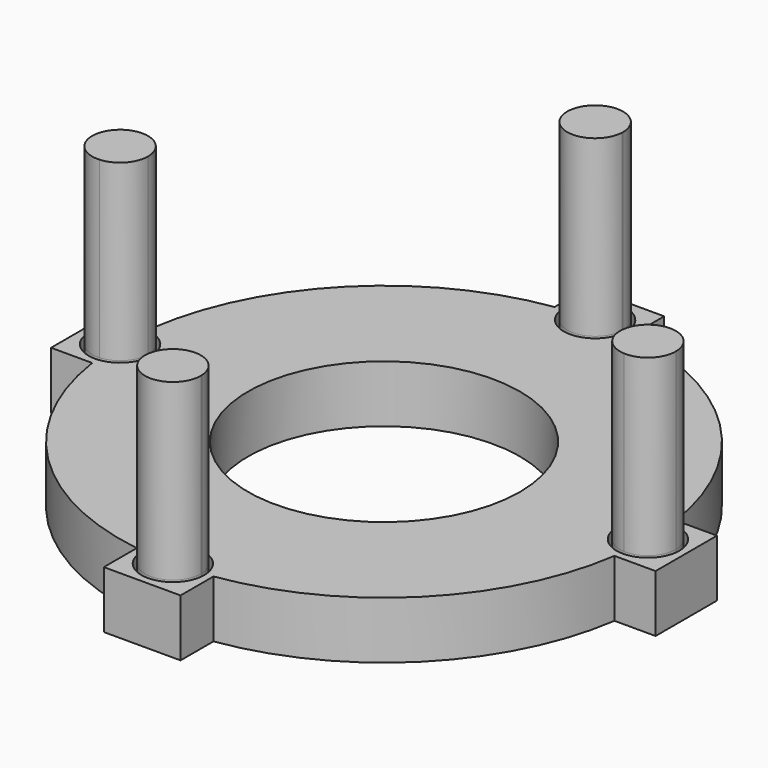
from build123d import *

# Parameters (mm, degrees)
F0_R     = 20
F0_R_2   = 19.5
F1_DEPTH = 8.2
F3_DEPTH = 25


# Not quite as in the source:
# - the program builds the solid bodies; features that only make, move or delete a surface that nothing else refers to are left out


with BuildPart() as f1:
    # F0 (on Top) → F1 (new body)
    with BuildSketch(Plane.XY):
        with BuildLine():
            ThreePointArc((37.5774613555, -4.492039968), (33.345, 0), (37.5774613555, 4.492039968))
            ThreePointArc((37.5774613555, 4.492039968), (37.5137215364, 4.9964709038), (37.4432106663, 5.5))
            Line((37.4432106663, 5.5), (32.345, 5.5))
            Line((32.345, 5.5), (32.345, -5.5))
            Line((32.345, -5.5), (37.4432106663, -5.5))
            ThreePointArc((37.4432106663, -5.5), (37.5137215364, -4.9964709038), (37.5774613555, -4.492039968))
        make_face()
        with BuildLine():
            ThreePointArc((37.4432106663, 5.5), (37.5137215364, 4.9964709038), (37.5774613555, 4.492039968))
            ThreePointArc((37.5774613555, 4.492039968), (40.9309420037, 3.2752041082), (42.345, 0))
            ThreePointArc((42.345, 0), (40.9309420037, -3.2752041082), (37.5774613555, -4.492039968))
            ThreePointArc((37.5774613555, -4.492039968), (37.5137215364, -4.9964709038), (37.4432106663, -5.5))
            Line((37.4432106663, -5.5), (43.345, -5.5))
            Line((43.345, -5.5), (43.345, 5.5))
            Line((43.345, 5.5), (37.4432106663, 5.5))
        make_face()
        with BuildLine():
            Line((32.345, 5.5), (37.4432106663, 5.5))
            ThreePointArc((37.4432106663, 5.5), (26.760456134, 26.760456134), (5.5, 37.4432106663))
            Line((5.5, 37.4432106663), (5.5, 32.345))
            Line((5.5, 32.345), (-5.5, 32.345))
            Line((-5.5, 32.345), (-5.5, 37.4432106663))
            ThreePointArc((-5.5, 37.4432106663), (-26.760456134, 26.760456134), (-37.4432106663, 5.5))
            Line((-37.4432106663, 5.5), (-32.345, 5.5))
            Line((-32.345, 5.5), (-32.345, -5.5))
            Line((-32.345, -5.5), (-37.4432106663, -5.5))
            ThreePointArc((-37.4432106663, -5.5), (-26.760456134, -26.760456134), (-5.5, -37.4432106663))
            Line((-5.5, -37.4432106663), (-5.5, -32.345))
            Line((-5.5, -32.345), (5.5, -32.345))
            Line((5.5, -32.345), (5.5, -37.4432106663))
            ThreePointArc((5.5, -37.4432106663), (26.760456134, -26.760456134), (37.4432106663, -5.5))
            Line((37.4432106663, -5.5), (32.345, -5.5))
            Line((32.345, -5.5), (32.345, 5.5))
        make_face()
        with BuildLine():
            ThreePointArc((23.3205760812, 16.9760053087), (27.4291454667, 8.9261416059), (28.845, 0))
            ThreePointArc((28.845, 0), (27.4291454667, -8.9261416059), (23.3205760812, -16.9760053087))
            ThreePointArc((23.3205760812, -16.9760053087), (24.483570121, -18.5134609029), (24.8964951033, -20.3964951033))
            ThreePointArc((24.8964951033, -20.3964951033), (21.9549873112, -24.6179998158), (16.9760053087, -23.3205760812))
            ThreePointArc((16.9760053087, -23.3205760812), (0, -28.845), (-16.9760053087, -23.3205760812))
            ThreePointArc((-16.9760053087, -23.3205760812), (-23.5784756187, -23.5784756187), (-23.3205760812, -16.9760053087))
            ThreePointArc((-23.3205760812, -16.9760053087), (-28.845, 0), (-23.3205760812, 16.9760053087))
            ThreePointArc((-23.3205760812, 16.9760053087), (-23.5784756187, 23.5784756187), (-16.9760053087, 23.3205760812))
            ThreePointArc((-16.9760053087, 23.3205760812), (0, 28.845), (16.9760053087, 23.3205760812))
            ThreePointArc((16.9760053087, 23.3205760812), (21.9549873112, 24.6179998158), (24.8964951033, 20.3964951033))
            ThreePointArc((24.8964951033, 20.3964951033), (24.483570121, 18.5134609029), (23.3205760812, 16.9760053087))
        make_face(mode=Mode.SUBTRACT)
        with BuildLine():
            Line((5.5, 32.345), (5.5, 37.4432106663))
            ThreePointArc((5.5, 37.4432106663), (4.9964709038, 37.5137215364), (4.492039968, 37.5774613555))
            ThreePointArc((4.492039968, 37.5774613555), (0, 33.345), (-4.492039968, 37.5774613555))
            ThreePointArc((-4.492039968, 37.5774613555), (-4.9964709038, 37.5137215364), (-5.5, 37.4432106663))
            Line((-5.5, 37.4432106663), (-5.5, 32.345))
            Line((-5.5, 32.345), (5.5, 32.345))
        make_face()
        with BuildLine():
            ThreePointArc((4.492039968, 37.5774613555), (4.9964709038, 37.5137215364), (5.5, 37.4432106663))
            Line((5.5, 37.4432106663), (5.5, 43.345))
            Line((5.5, 43.345), (-5.5, 43.345))
            Line((-5.5, 43.345), (-5.5, 37.4432106663))
            ThreePointArc((-5.5, 37.4432106663), (-4.9964709038, 37.5137215364), (-4.492039968, 37.5774613555))
            ThreePointArc((-4.492039968, 37.5774613555), (-0.1338285175, 42.3430095518), (4.5, 37.845))
            ThreePointArc((4.5, 37.845), (4.4980095518, 37.7111714825), (4.492039968, 37.5774613555))
        make_face()
        with BuildLine():
            Line((5.5, -43.345), (5.5, -37.4432106663))
            ThreePointArc((5.5, -37.4432106663), (4.9964709038, -37.5137215364), (4.492039968, -37.5774613555))
            ThreePointArc((4.492039968, -37.5774613555), (4.4980095518, -37.7111714825), (4.5, -37.845))
            ThreePointArc((4.5, -37.845), (-0.1338285175, -42.3430095518), (-4.492039968, -37.5774613555))
            ThreePointArc((-4.492039968, -37.5774613555), (-4.9964709038, -37.5137215364), (-5.5, -37.4432106663))
            Line((-5.5, -37.4432106663), (-5.5, -43.345))
            Line((-5.5, -43.345), (5.5, -43.345))
        make_face()
        with BuildLine():
            ThreePointArc((4.492039968, -37.5774613555), (4.9964709038, -37.5137215364), (5.5, -37.4432106663))
            Line((5.5, -37.4432106663), (5.5, -32.345))
            Line((5.5, -32.345), (-5.5, -32.345))
            Line((-5.5, -32.345), (-5.5, -37.4432106663))
            ThreePointArc((-5.5, -37.4432106663), (-4.9964709038, -37.5137215364), (-4.492039968, -37.5774613555))
            ThreePointArc((-4.492039968, -37.5774613555), (0, -33.345), (4.492039968, -37.5774613555))
        make_face()
        with BuildLine():
            Line((-32.345, 5.5), (-37.4432106663, 5.5))
            ThreePointArc((-37.4432106663, 5.5), (-37.5137215364, 4.9964709038), (-37.5774613555, 4.492039968))
            ThreePointArc((-37.5774613555, 4.492039968), (-34.5697958918, 3.0859420037), (-33.345, 0))
            ThreePointArc((-33.345, 0), (-34.5697958918, -3.0859420037), (-37.5774613555, -4.492039968))
            ThreePointArc((-37.5774613555, -4.492039968), (-37.5137215364, -4.9964709038), (-37.4432106663, -5.5))
            Line((-37.4432106663, -5.5), (-32.345, -5.5))
            Line((-32.345, -5.5), (-32.345, 5.5))
        make_face()
        with BuildLine():
            ThreePointArc((-37.5774613555, 4.492039968), (-37.5137215364, 4.9964709038), (-37.4432106663, 5.5))
            Line((-37.4432106663, 5.5), (-43.345, 5.5))
            Line((-43.345, 5.5), (-43.345, -5.5))
            Line((-43.345, -5.5), (-37.4432106663, -5.5))
            ThreePointArc((-37.4432106663, -5.5), (-37.5137215364, -4.9964709038), (-37.5774613555, -4.492039968))
            ThreePointArc((-37.5774613555, -4.492039968), (-42.345, 0), (-37.5774613555, 4.492039968))
        make_face()
        with BuildLine():
            ThreePointArc((-23.3205760812, 16.9760053087), (-20.3964951033, 20.3964951033), (-16.9760053087, 23.3205760812))
            ThreePointArc((-16.9760053087, 23.3205760812), (-23.5784756187, 23.5784756187), (-23.3205760812, 16.9760053087))
        make_face()
        with BuildLine():
            ThreePointArc((16.9760053087, 23.3205760812), (20.3964951033, 20.3964951033), (23.3205760812, 16.9760053087))
            ThreePointArc((23.3205760812, 16.9760053087), (24.483570121, 18.5134609029), (24.8964951033, 20.3964951033))
            ThreePointArc((24.8964951033, 20.3964951033), (21.9549873112, 24.6179998158), (16.9760053087, 23.3205760812))
        make_face()
        with BuildLine():
            ThreePointArc((24.8964951033, -20.3964951033), (24.483570121, -18.5134609029), (23.3205760812, -16.9760053087))
            ThreePointArc((23.3205760812, -16.9760053087), (20.3964951033, -20.3964951033), (16.9760053087, -23.3205760812))
            ThreePointArc((16.9760053087, -23.3205760812), (21.9549873112, -24.6179998158), (24.8964951033, -20.3964951033))
        make_face()
        with BuildLine():
            ThreePointArc((-23.3205760812, -16.9760053087), (-23.5784756187, -23.5784756187), (-16.9760053087, -23.3205760812))
            ThreePointArc((-16.9760053087, -23.3205760812), (-20.3964951033, -20.3964951033), (-23.3205760812, -16.9760053087))
        make_face()
        with BuildLine():
            ThreePointArc((23.3205760812, -16.9760053087), (27.4291454667, -8.9261416059), (28.845, 0))
            ThreePointArc((28.845, 0), (27.4291454667, 8.9261416059), (23.3205760812, 16.9760053087))
            ThreePointArc((23.3205760812, 16.9760053087), (17.214514588, 17.214514588), (16.9760053087, 23.3205760812))
            ThreePointArc((16.9760053087, 23.3205760812), (0, 28.845), (-16.9760053087, 23.3205760812))
            ThreePointArc((-16.9760053087, 23.3205760812), (-16.1749903908, 21.9549873112), (-15.8964951033, 20.3964951033))
            ThreePointArc((-15.8964951033, 20.3964951033), (-18.5134609029, 16.3094200856), (-23.3205760812, 16.9760053087))
            ThreePointArc((-23.3205760812, 16.9760053087), (-28.845, 0), (-23.3205760812, -16.9760053087))
            ThreePointArc((-23.3205760812, -16.9760053087), (-18.5134609029, -16.3094200856), (-15.8964951033, -20.3964951033))
            ThreePointArc((-15.8964951033, -20.3964951033), (-16.1749903908, -21.9549873112), (-16.9760053087, -23.3205760812))
            ThreePointArc((-16.9760053087, -23.3205760812), (0, -28.845), (16.9760053087, -23.3205760812))
            ThreePointArc((16.9760053087, -23.3205760812), (17.214514588, -17.214514588), (23.3205760812, -16.9760053087))
        make_face()
        Circle(F0_R, mode=Mode.SUBTRACT)
        with BuildLine():
            ThreePointArc((16.9760053087, -23.3205760812), (20.3964951033, -20.3964951033), (23.3205760812, -16.9760053087))
            ThreePointArc((23.3205760812, -16.9760053087), (17.214514588, -17.214514588), (16.9760053087, -23.3205760812))
        make_face()
        with BuildLine():
            ThreePointArc((16.9760053087, 23.3205760812), (17.214514588, 17.214514588), (23.3205760812, 16.9760053087))
            ThreePointArc((23.3205760812, 16.9760053087), (20.3964951033, 20.3964951033), (16.9760053087, 23.3205760812))
        make_face()
        with BuildLine():
            ThreePointArc((-15.8964951033, 20.3964951033), (-16.1749903908, 21.9549873112), (-16.9760053087, 23.3205760812))
            ThreePointArc((-16.9760053087, 23.3205760812), (-20.3964951033, 20.3964951033), (-23.3205760812, 16.9760053087))
            ThreePointArc((-23.3205760812, 16.9760053087), (-18.5134609029, 16.3094200856), (-15.8964951033, 20.3964951033))
        make_face()
        with BuildLine():
            ThreePointArc((-23.3205760812, -16.9760053087), (-20.3964951033, -20.3964951033), (-16.9760053087, -23.3205760812))
            ThreePointArc((-16.9760053087, -23.3205760812), (-16.1749903908, -21.9549873112), (-15.8964951033, -20.3964951033))
            ThreePointArc((-15.8964951033, -20.3964951033), (-18.5134609029, -16.3094200856), (-23.3205760812, -16.9760053087))
        make_face()
        Circle(F0_R)
        Circle(F0_R_2, mode=Mode.SUBTRACT)
    extrude(amount=F1_DEPTH)


with BuildPart() as f1b:
    # F0 (on Top) → F1, piece 2 (new body)
    with BuildSketch(Plane.XY):
        with BuildLine():
            ThreePointArc((-37.6336114414, -3.9944104543), (-37.845, 0), (-37.6336114414, 3.9944104543))
            ThreePointArc((-37.6336114414, 3.9944104543), (-41.845, 0), (-37.6336114414, -3.9944104543))
        make_face()
        with BuildLine():
            ThreePointArc((-33.845, 0), (-34.9427978848, 2.7526755862), (-37.6336114414, 3.9944104543))
            ThreePointArc((-37.6336114414, 3.9944104543), (-37.845, 0), (-37.6336114414, -3.9944104543))
            ThreePointArc((-37.6336114414, -3.9944104543), (-34.9427978848, -2.7526755862), (-33.845, 0))
        make_face()
    extrude(amount=F1_DEPTH)


with BuildPart() as f1c:
    # F0 (on Top) → F1, piece 3 (new body)
    with BuildSketch(Plane.XY):
        with BuildLine():
            ThreePointArc((-3.9944104543, 37.6336114414), (0, 37.845), (3.9944104543, 37.6336114414))
            ThreePointArc((3.9944104543, 37.6336114414), (3.9986023694, 37.7392687774), (4, 37.845))
            ThreePointArc((4, 37.845), (-0.1057312226, 41.8436023694), (-3.9944104543, 37.6336114414))
        make_face()
        with BuildLine():
            ThreePointArc((-3.9944104543, 37.6336114414), (0, 33.845), (3.9944104543, 37.6336114414))
            ThreePointArc((3.9944104543, 37.6336114414), (0, 37.845), (-3.9944104543, 37.6336114414))
        make_face()
    extrude(amount=F1_DEPTH)


with BuildPart() as f1d:
    # F0 (on Top) → F1, piece 4 (new body)
    with BuildSketch(Plane.XY):
        with BuildLine():
            ThreePointArc((37.6336114414, -3.9944104543), (37.7921159106, -2), (37.845, 0))
            ThreePointArc((37.845, 0), (37.7921159106, 2), (37.6336114414, 3.9944104543))
            ThreePointArc((37.6336114414, 3.9944104543), (33.845, 0), (37.6336114414, -3.9944104543))
        make_face()
        with BuildLine():
            ThreePointArc((37.6336114414, 3.9944104543), (37.7921159106, 2), (37.845, 0))
            ThreePointArc((37.845, 0), (37.7921159106, -2), (37.6336114414, -3.9944104543))
            ThreePointArc((37.6336114414, -3.9944104543), (40.5976755862, -2.9022021152), (41.845, 0))
            ThreePointArc((41.845, 0), (40.5976755862, 2.9022021152), (37.6336114414, 3.9944104543))
        make_face()
    extrude(amount=F1_DEPTH)


with BuildPart() as f1e:
    # F0 (on Top) → F1, piece 5 (new body)
    with BuildSketch(Plane.XY):
        with BuildLine():
            ThreePointArc((-3.9944104543, -37.6336114414), (0, -37.845), (3.9944104543, -37.6336114414))
            ThreePointArc((3.9944104543, -37.6336114414), (0, -33.845), (-3.9944104543, -37.6336114414))
        make_face()
        with BuildLine():
            ThreePointArc((4, -37.845), (3.9986023694, -37.7392687774), (3.9944104543, -37.6336114414))
            ThreePointArc((3.9944104543, -37.6336114414), (0, -37.845), (-3.9944104543, -37.6336114414))
            ThreePointArc((-3.9944104543, -37.6336114414), (-0.1057312226, -41.8436023694), (4, -37.845))
        make_face()
    extrude(amount=F1_DEPTH)


with BuildPart() as f3:
    # F3 (new): a face of the model
    f3_faces = [f1c.part.faces().sort_by_distance(p)[0] for p in [
        (0, 37.845, 8.2),
    ]]
    extrude(f3_faces, amount=F3_DEPTH)


with BuildPart() as f3b:
    # F3#2 (new): a face of the model
    f3_2_faces = [f1b.part.faces().sort_by_distance(p)[0] for p in [
        (-37.845, 0, 8.2),
    ]]
    extrude(f3_2_faces, amount=F3_DEPTH)


with BuildPart() as f3c:
    # F3#3 (new): a face of the model
    f3_3_faces = [f1d.part.faces().sort_by_distance(p)[0] for p in [
        (37.845, 0, 8.2),
    ]]
    extrude(f3_3_faces, amount=F3_DEPTH)


with BuildPart() as f3d:
    # F3#4 (new): a face of the model
    f3_4_faces = [f1e.part.faces().sort_by_distance(p)[0] for p in [
        (0, -37.845, 8.2),
    ]]
    extrude(f3_4_faces, amount=F3_DEPTH)


solid = Compound([f1.part, f1b.part, f1c.part, f1d.part, f1e.part, f3.part, f3b.part, f3c.part, f3d.part])
